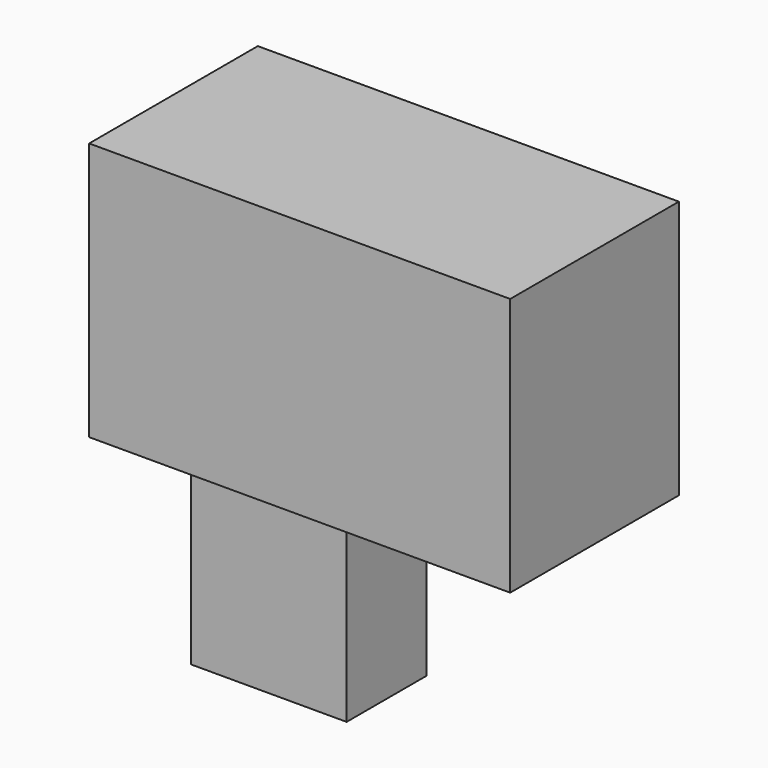
from build123d import *

# Parameters (mm, degrees)
F0_W     = 52.2512793541
F0_H     = 32.0903435349
F1_DEPTH = 26.162
F2_W     = 19.282985013
F2_H     = 12.3756476678
F3_DEPTH = 25.4


# Not quite as in the source:
# - a feature names something its author has since deleted; it is built from what else it names


with BuildPart() as f1:
    # F0 (on Front) → F1 (new body)
    with BuildSketch(Plane.XZ):
        with Locations((26.125639677, 16.0451717675)):
            Rectangle(F0_W, F0_H)
    extrude(amount=F1_DEPTH)

    # F2 (on face) → F3 (join)
    with BuildSketch(Plane(origin=(0, 0, 0), x_dir=(1, 0, 0), z_dir=(0, 0, -1))):
        with Locations((16.692733625, 12.9512592684)):
            Rectangle(F2_W, F2_H)
    extrude(amount=F3_DEPTH)


solid = f1.part
